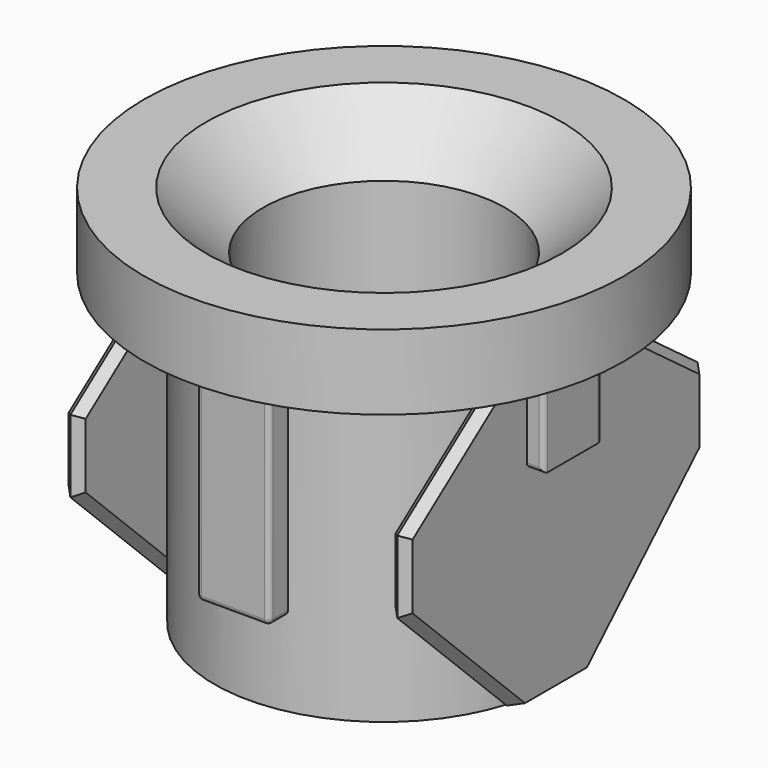
from build123d import *

# Parameters (mm, degrees)
F0_R          = 3.5
F0_R_2        = 3.1
F1_DEPTH      = 2.1
F2_R          = 3.5
F2_R_2        = 3.1
F2_R_3        = 2.5
F3_DEPTH      = 4.24
F4_R          = 4.95
F4_R_2        = 3.5
F4_R_3        = 2.5
F5_DEPTH      = 1.55
F6_SIZE       = 1.175
F8_DEPTH      = 4.6
F9_DEPTH      = 2.09
F10_R         = 0.1
F11_W         = 0.35
F11_H         = 3.875
F12_DEPTH     = 6.34
F14_DEPTH     = 0.38076
F16_T1_DEPTH  = 4.8355972722
F16_T3_DEPTH  = 2.4000890458
F16_T5_DEPTH  = 4.8355972722
F16_T10_DEPTH = 4.4201210059
F16_T15_DEPTH = 4.638323219
F16_S16_R     = 3.5
F16_T17_DEPTH = 4
F16_T21_DEPTH = 4.2769316216
F16_S23_R     = 3.5
F16_T24_DEPTH = 4
F16_T28_DEPTH = 4.638323219
F16_S29_R     = 3.5
F16_T30_DEPTH = 4
F16_T34_DEPTH = 4.4201210059
F16_T39_DEPTH = 4.2769316216
F16_S41_R     = 3.5
F16_T42_DEPTH = 4
F16_T46_DEPTH = 4.2769316216
F16_S48_R     = 3.5
F16_T49_DEPTH = 4
F16_T53_DEPTH = 4.4201210059
F16_T58_DEPTH = 4.638323219
F16_S59_R     = 3.5
F16_T60_DEPTH = 4
F16_T64_DEPTH = 4.4201210059
F16_T69_DEPTH = 4.2769316216
F16_S71_R     = 3.5
F16_T72_DEPTH = 4
F16_T76_DEPTH = 4.638323219
F16_S77_R     = 3.5
F16_T78_DEPTH = 4


# Not quite as in the source:
# - a fillet or chamfer that OpenCascade refuses, or shapes differently, is made with other operations: its cross-section is extruded or revolved along the edge and cut away or added


with BuildPart() as f1:
    # F0 (on Top) → F1 (new body)
    with BuildSketch(Plane.XY):
        Circle(F0_R)
        Circle(F0_R_2, mode=Mode.SUBTRACT)
    extrude(amount=F1_DEPTH)

    # F2 (on face) → F3 (join)
    with BuildSketch(Plane.XY.offset(2.1)):
        Circle(F2_R)
        Circle(F2_R_2, mode=Mode.SUBTRACT)
        Circle(F2_R_2)
        Circle(F2_R_3, mode=Mode.SUBTRACT)
    extrude(amount=F3_DEPTH)

    # F4 (on face) → F5 (join)
    with BuildSketch(Plane.XY.offset(6.34)):
        Circle(F4_R)
        Circle(F4_R_2, mode=Mode.SUBTRACT)
        Circle(F4_R_2)
        Circle(F4_R_3, mode=Mode.SUBTRACT)
    extrude(amount=F5_DEPTH)

    # F6
    f6_edges = [f1.edges().sort_by_distance(p)[0] for p in [
        (-2.5, 0, 7.89),
    ]]
    chamfer(f6_edges, length=F6_SIZE)

    # F7 (on face) → F8 (join)
    with BuildSketch(Plane(origin=(0, 0, 6.34), x_dir=(1, 0, 0), z_dir=(0, 0, -1))):
        with BuildLine():
            Line((-0.75, -3.9), (0, -3.9))
            Line((0, -3.9), (0.75, -3.9))
            Line((0.75, -3.9), (0.75, -3.4186985828))
            ThreePointArc((0.75, -3.4186985828), (0, -3.5), (-0.75, -3.4186985828))
            Line((-0.75, -3.4186985828), (-0.75, -3.9))
        make_face()
        with BuildLine():
            Line((-0.75, 3.9), (-0.75, 3.4186985828))
            ThreePointArc((-0.75, 3.4186985828), (0, 3.5), (0.75, 3.4186985828))
            Line((0.75, 3.4186985828), (0.75, 3.9))
            Line((0.75, 3.9), (0, 3.9))
            Line((0, 3.9), (-0.75, 3.9))
        make_face()
    extrude(amount=F8_DEPTH)

    # F7 (on face) → F9 (join)
    with BuildSketch(Plane(origin=(0, 0, 6.34), x_dir=(1, 0, 0), z_dir=(0, 0, -1))):
        with BuildLine():
            Line((-3.9, -0.75), (-3.4186985828, -0.75))
            ThreePointArc((-3.4186985828, -0.75), (-3.5, 0), (-3.4186985828, 0.75))
            Line((-3.4186985828, 0.75), (-3.9, 0.75))
            Line((-3.9, 0.75), (-3.9, 0))
            Line((-3.9, 0), (-3.9, -0.75))
        make_face()
        with BuildLine():
            ThreePointArc((3.5, 0), (3.4796152833, -0.3771968718), (3.4186985828, -0.75))
            Line((3.4186985828, -0.75), (3.9, -0.75))
            Line((3.9, -0.75), (3.9, 0))
            Line((3.9, 0), (3.9, 0.75))
            Line((3.9, 0.75), (3.4186985828, 0.75))
            ThreePointArc((3.4186985828, 0.75), (3.4796152833, 0.3771968718), (3.5, 0))
        make_face()
    extrude(amount=F9_DEPTH)

    # F10
    f10_edges = [f1.edges().sort_by_distance(p)[0] for p in [
        (0.75, 3.659349, 1.74),
        (0, 3.9, 1.74),
        (0.75, 3.9, 4.04),
        (3.659349, 0.75, 4.25),
        (3.9, 0.75, 5.295),
        (3.659349, -0.75, 4.25),
        (3.9, -0.75, 5.295),
        (0, -3.9, 1.74),
        (0.75, -3.9, 4.04),
        (0.75, -3.659349, 1.74),
        (-0.75, -3.9, 4.04),
        (-0.75, -3.659349, 1.74),
        (-3.9, -0.75, 5.295),
        (-3.9, 0, 4.25),
        (-3.9, 0.75, 5.295),
        (-3.659349, 0.75, 4.25),
        (-3.659349, -0.75, 4.25),
        (-0.75, 3.9, 4.04),
        (-0.75, 3.659349, 1.74),
    ]]
    fillet(f10_edges, radius=F10_R)

    # F11 (on face) → F12 (join)
    with BuildSketch(Plane(origin=(0, 0, 6.34), x_dir=(1, 0, 0), z_dir=(0, 0, -1))):
        with Locations((3.375, 1.9375)):
            Rectangle(F11_W, F11_H)
        with Locations((3.375, -1.9375)):
            Rectangle(F11_W, F11_H)
    extrude(amount=F12_DEPTH)

    # F13 (on face) → F14 (cut)
    with BuildSketch(Plane.YZ.offset(3.55)):
        Polygon((-3.875, 6.34), (-3.875, 4.24), (-1.05, 6.34), (-3.4496376621, 6.34), align=None)
        Polygon((1.05, 6.34), (3.875, 4.24), (3.875, 6.34), (3.4496376621, 6.34), align=None)
        Polygon((3.875, 2.74), (1.05, 0), (3.875, 0), align=None)
        Polygon((-1.05, 0), (-3.875, 2.74), (-3.875, 0), align=None)
    extrude(amount=-F14_DEPTH, mode=Mode.SUBTRACT)

    # F15: F1 across plane


with BuildPart() as f1_1:
    add(f1.part)
    add(f1.part.mirror(Plane.YZ))

    # F16: chamfer of 0.175 on 24 edges, made by hand

    # F16_s2 → F16_t1 (cut)
    with BuildSketch(Plane(origin=(0, 3.6890864967, 3.5780874339), x_dir=(1, 0, 0), z_dir=(0, -0.7178234265, -0.6962251995))):
        Polygon((-3.375, -0.7310364595), (-3.55, -0.5560364595), (-3.55, -0.7310364595), align=None)
        Polygon((3.375, -0.7310364595), (3.55, -0.5560364595), (3.55, -0.7310364595), align=None)
    extrude(amount=F16_T1_DEPTH, mode=Mode.SUBTRACT)

    # F16_s4 → F16_t3 (cut)
    with BuildSketch(Plane.XY.offset(2.2899554771)):
        Polygon((-3.375, 3.875), (-3.55, 3.7), (-3.55, 3.875), align=None)
        Polygon((-3.2, 3.7), (-3.375, 3.875), (-3.2, 3.875), align=None)
        Polygon((-3.375, -3.875), (-3.55, -3.7), (-3.55, -3.875), align=None)
        Polygon((-3.2, -3.7), (-3.375, -3.875), (-3.2, -3.875), align=None)
        Polygon((3.2, -3.7), (3.375, -3.875), (3.2, -3.875), align=None)
        Polygon((3.375, -3.875), (3.55, -3.7), (3.55, -3.875), align=None)
        Polygon((3.375, 3.875), (3.55, 3.7), (3.55, 3.875), align=None)
        Polygon((3.375, 3.875), (3.2, 3.7), (3.2, 3.875), align=None)
    extrude(amount=F16_T3_DEPTH, mode=Mode.SUBTRACT)

    # F16_s6 → F16_t5 (cut)
    with BuildSketch(Plane(origin=(0, -0.2179814937, 0.2114227585), x_dir=(1, 0, 0), z_dir=(0, -0.7178234265, 0.6962251995))):
        Polygon((-3.375, -0.7310364595), (-3.55, -0.5560364595), (-3.55, -0.7310364595), align=None)
        Polygon((3.375, -0.7310364595), (3.55, -0.5560364595), (3.55, -0.7310364595), align=None)
    extrude(amount=F16_T5_DEPTH, mode=Mode.SUBTRACT)


with BuildPart() as f16_tool8:
    # F16_s9 → F16_t10 (new body)
    with BuildSketch(Plane(origin=(0, -2.7204178255, 2.0222574986), x_dir=(1, 0, 0), z_dir=(0, 0.8025495314, -0.5965854924))):
        Polygon((-3.375, -5.7145787959), (-3.55, -5.5395787959), (-3.55, -5.7145787959), align=None)
    extrude(amount=F16_T10_DEPTH)

    split(bisect_by=Plane.XY.offset(6.34), keep=Keep.BOTTOM)


with BuildPart() as f1_2:
    add(f1_1.part)

    # F16_t7: cut F16_tool8
    add(f16_tool8.part, mode=Mode.SUBTRACT)


with BuildPart() as f16_tool13:
    # F16_s14 → F16_t15 (new body)
    with BuildSketch(Plane(origin=(0, 3.6890864967, 3.5780874339), x_dir=(1, 0, 0), z_dir=(0, -0.7178234265, -0.6962251995))):
        Polygon((-3.2, -0.5560364595), (-3.375, -0.7310364595), (-3.2, -0.7310364595), align=None)
    extrude(amount=F16_T15_DEPTH)

    # F16_s16 → F16_t17 (cut, symmetric)
    with BuildSketch(Plane.XY.offset(1.5)):
        Circle(F16_S16_R)
    extrude(amount=F16_T17_DEPTH, both=True, mode=Mode.SUBTRACT)


with BuildPart() as f1_3:
    add(f1_2.part)

    # F16_t12: cut F16_tool13
    add(f16_tool13.part, mode=Mode.SUBTRACT)


with BuildPart() as f16_tool19:
    # F16_s20 → F16_t21 (new body)
    with BuildSketch(Plane(origin=(0, -2.6055012523, 1.9368327893), x_dir=(1, 0, 0), z_dir=(0, 0.8025495314, -0.5965854924))):
        Polygon((-3.375, -5.7145787959), (-3.2, -5.5395787959), (-3.2, -5.7145787959), align=None)
    extrude(amount=F16_T21_DEPTH)

    split(bisect_by=Plane.XY.offset(6.34), keep=Keep.BOTTOM)

    # F16_s23 → F16_t24 (cut, symmetric)
    with BuildSketch(Plane.XY.offset(5.2)):
        Circle(F16_S23_R)
    extrude(amount=F16_T24_DEPTH, both=True, mode=Mode.SUBTRACT)


with BuildPart() as f1_4:
    add(f1_3.part)

    # F16_t18: cut F16_tool19
    add(f16_tool19.part, mode=Mode.SUBTRACT)


with BuildPart() as f16_tool26:
    # F16_s27 → F16_t28 (new body)
    with BuildSketch(Plane(origin=(0, -0.3595894305, 0.3487699255), x_dir=(1, 0, 0), z_dir=(0, -0.7178234265, 0.6962251995))):
        Polygon((-3.375, -0.7310364595), (-3.2, -0.5560364595), (-3.2, -0.7310364595), align=None)
    extrude(amount=F16_T28_DEPTH)

    # F16_s29 → F16_t30 (cut, symmetric)
    with BuildSketch(Plane.XY.offset(1.5)):
        Circle(F16_S29_R)
    extrude(amount=F16_T30_DEPTH, both=True, mode=Mode.SUBTRACT)


with BuildPart() as f1_5:
    add(f1_4.part)

    # F16_t25: cut F16_tool26
    add(f16_tool26.part, mode=Mode.SUBTRACT)


with BuildPart() as f16_tool32:
    # F16_s33 → F16_t34 (new body)
    with BuildSketch(Plane(origin=(0, -0.8269482164, -0.6147225679), x_dir=(1, 0, 0), z_dir=(0, 0.8025495314, 0.5965854924))):
        Polygon((-3.55, -5.5395787959), (-3.375, -5.7145787959), (-3.55, -5.7145787959), align=None)
    extrude(amount=F16_T34_DEPTH)

    split(bisect_by=Plane.XY.offset(6.34), keep=Keep.BOTTOM)


with BuildPart() as f1_6:
    add(f1_5.part)

    # F16_t31: cut F16_tool32
    add(f16_tool32.part, mode=Mode.SUBTRACT)


with BuildPart() as f16_tool37:
    # F16_s38 → F16_t39 (new body)
    with BuildSketch(Plane(origin=(0, -0.8269482164, -0.6147225679), x_dir=(1, 0, 0), z_dir=(0, 0.8025495314, 0.5965854924))):
        Polygon((-3.2, -5.5395787959), (-3.375, -5.7145787959), (-3.2, -5.7145787959), align=None)
    extrude(amount=F16_T39_DEPTH)

    split(bisect_by=Plane.XY.offset(6.34), keep=Keep.BOTTOM)

    # F16_s41 → F16_t42 (cut, symmetric)
    with BuildSketch(Plane.XY.offset(5.2)):
        Circle(F16_S41_R)
    extrude(amount=F16_T42_DEPTH, both=True, mode=Mode.SUBTRACT)


with BuildPart() as f1_7:
    add(f1_6.part)

    # F16_t36: cut F16_tool37
    add(f16_tool37.part, mode=Mode.SUBTRACT)


with BuildPart() as f16_tool44:
    # F16_s45 → F16_t46 (new body)
    with BuildSketch(Plane(origin=(0, -0.8269482164, -0.6147225679), x_dir=(1, 0, 0), z_dir=(0, 0.8025495314, 0.5965854924))):
        Polygon((3.2, -5.5395787959), (3.375, -5.7145787959), (3.2, -5.7145787959), align=None)
    extrude(amount=F16_T46_DEPTH)

    split(bisect_by=Plane.XY.offset(6.34), keep=Keep.BOTTOM)

    # F16_s48 → F16_t49 (cut, symmetric)
    with BuildSketch(Plane.XY.offset(5.2)):
        Circle(F16_S48_R)
    extrude(amount=F16_T49_DEPTH, both=True, mode=Mode.SUBTRACT)


with BuildPart() as f1_8:
    add(f1_7.part)

    # F16_t43: cut F16_tool44
    add(f16_tool44.part, mode=Mode.SUBTRACT)


with BuildPart() as f16_tool51:
    # F16_s52 → F16_t53 (new body)
    with BuildSketch(Plane(origin=(0, -0.8269482164, -0.6147225679), x_dir=(1, 0, 0), z_dir=(0, 0.8025495314, 0.5965854924))):
        Polygon((3.375, -5.7145787959), (3.55, -5.5395787959), (3.55, -5.7145787959), align=None)
    extrude(amount=F16_T53_DEPTH)

    split(bisect_by=Plane.XY.offset(6.34), keep=Keep.BOTTOM)


with BuildPart() as f1_9:
    add(f1_8.part)

    # F16_t50: cut F16_tool51
    add(f16_tool51.part, mode=Mode.SUBTRACT)


with BuildPart() as f16_tool56:
    # F16_s57 → F16_t58 (new body)
    with BuildSketch(Plane(origin=(0, -0.3595894305, 0.3487699255), x_dir=(1, 0, 0), z_dir=(0, -0.7178234265, 0.6962251995))):
        Polygon((3.375, -0.7310364595), (3.2, -0.5560364595), (3.2, -0.7310364595), align=None)
    extrude(amount=F16_T58_DEPTH)

    # F16_s59 → F16_t60 (cut, symmetric)
    with BuildSketch(Plane.XY.offset(1.5)):
        Circle(F16_S59_R)
    extrude(amount=F16_T60_DEPTH, both=True, mode=Mode.SUBTRACT)


with BuildPart() as f1_10:
    add(f1_9.part)

    # F16_t55: cut F16_tool56
    add(f16_tool56.part, mode=Mode.SUBTRACT)


with BuildPart() as f16_tool62:
    # F16_s63 → F16_t64 (new body)
    with BuildSketch(Plane(origin=(0, -2.7204178255, 2.0222574986), x_dir=(1, 0, 0), z_dir=(0, 0.8025495314, -0.5965854924))):
        Polygon((3.55, -5.5395787959), (3.375, -5.7145787959), (3.55, -5.7145787959), align=None)
    extrude(amount=F16_T64_DEPTH)

    split(bisect_by=Plane.XY.offset(6.34), keep=Keep.BOTTOM)


with BuildPart() as f1_11:
    add(f1_10.part)

    # F16_t61: cut F16_tool62
    add(f16_tool62.part, mode=Mode.SUBTRACT)


with BuildPart() as f16_tool67:
    # F16_s68 → F16_t69 (new body)
    with BuildSketch(Plane(origin=(0, -2.6055012523, 1.9368327893), x_dir=(1, 0, 0), z_dir=(0, 0.8025495314, -0.5965854924))):
        Polygon((3.2, -5.5395787959), (3.375, -5.7145787959), (3.2, -5.7145787959), align=None)
    extrude(amount=F16_T69_DEPTH)

    split(bisect_by=Plane.XY.offset(6.34), keep=Keep.BOTTOM)

    # F16_s71 → F16_t72 (cut, symmetric)
    with BuildSketch(Plane.XY.offset(5.2)):
        Circle(F16_S71_R)
    extrude(amount=F16_T72_DEPTH, both=True, mode=Mode.SUBTRACT)


with BuildPart() as f1_12:
    add(f1_11.part)

    # F16_t66: cut F16_tool67
    add(f16_tool67.part, mode=Mode.SUBTRACT)


with BuildPart() as f16_tool74:
    # F16_s75 → F16_t76 (new body)
    with BuildSketch(Plane(origin=(0, 3.6890864967, 3.5780874339), x_dir=(1, 0, 0), z_dir=(0, -0.7178234265, -0.6962251995))):
        Polygon((3.375, -0.7310364595), (3.2, -0.5560364595), (3.2, -0.7310364595), align=None)
    extrude(amount=F16_T76_DEPTH)

    # F16_s77 → F16_t78 (cut, symmetric)
    with BuildSketch(Plane.XY.offset(1.5)):
        Circle(F16_S77_R)
    extrude(amount=F16_T78_DEPTH, both=True, mode=Mode.SUBTRACT)


with BuildPart() as f1_13:
    add(f1_12.part)

    # F16_t73: cut F16_tool74
    add(f16_tool74.part, mode=Mode.SUBTRACT)


solid = f1_13.part
